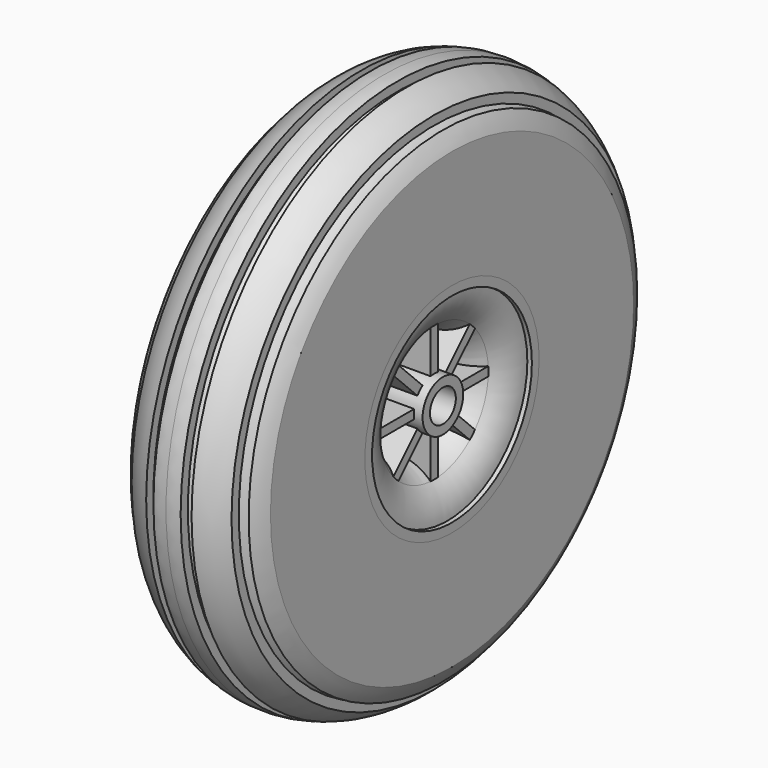
from build123d import *

# Parameters (mm, degrees)
F2_DEPTH = 0.635
F3_COUNT = 8
F3_ANGLE = 315


with BuildPart() as f1:
    # F0 (on Top) → F1 (revolve)
    with BuildSketch(Plane.XY):
        with BuildLine():
            Line((-8.255, 2.2606), (0, 2.2606))
            Line((0, 2.2606), (8.255, 2.2606))
            Line((8.255, 2.2606), (8.255, 3.556))
            Line((8.255, 3.556), (7.0301280605, 3.556))
            Line((7.0301280605, 3.556), (7.0301280605, 2.9083))
            Line((7.0301280605, 2.9083), (1.9207453588, 2.9083))
            Line((1.9207453588, 2.9083), (1.9207453588, 9.508256995))
            Line((1.9207453588, 9.508256995), (7.0301280605, 9.4798719395))
            ThreePointArc((7.0301280605, 9.4798719395), (8.4066350314, 11.5399602045), (8.89, 13.97))
            Line((8.89, 13.97), (9.525, 13.97))
            Line((9.525, 13.97), (9.525, 15.24))
            Line((9.525, 15.24), (8.255, 15.24))
            Line((8.255, 15.24), (8.255, 14.605))
            Line((8.255, 14.605), (0, 14.605))
            Line((0, 14.605), (-8.255, 14.605))
            Line((-8.255, 14.605), (-8.255, 15.24))
            Line((-8.255, 15.24), (-9.525, 15.24))
            Line((-9.525, 15.24), (-9.525, 13.97))
            Line((-9.525, 13.97), (-8.89, 13.97))
            ThreePointArc((-8.89, 13.97), (-8.4066350314, 11.5399602045), (-7.0301280605, 9.4798719395))
            Line((-7.0301280605, 9.4798719395), (-1.9207453588, 9.508256995))
            Line((-1.9207453588, 9.508256995), (-1.9207453588, 2.9083))
            Line((-1.9207453588, 2.9083), (-7.0301280605, 2.9083))
            Line((-7.0301280605, 2.9083), (-7.0301280605, 3.556))
            Line((-7.0301280605, 3.556), (-8.255, 3.556))
            Line((-8.255, 3.556), (-8.255, 2.2606))
        make_face()
        with BuildLine():
            Line((7.0301280605, 2.9083), (7.0301280605, 3.556))
            Line((7.0301280605, 3.556), (2.54, 3.556))
            Line((2.54, 3.556), (2.54, 7.62))
            ThreePointArc((2.54, 7.62), (4.9700397955, 8.1033649686), (7.0301280605, 9.4798719395))
            Line((7.0301280605, 9.4798719395), (1.9207453588, 9.508256995))
            Line((1.9207453588, 9.508256995), (1.9207453588, 2.9083))
            Line((1.9207453588, 2.9083), (7.0301280605, 2.9083))
        make_face()
        with BuildLine():
            Line((-2.54, 3.556), (-7.0301280605, 3.556))
            Line((-7.0301280605, 3.556), (-7.0301280605, 2.9083))
            Line((-7.0301280605, 2.9083), (-1.9207453588, 2.9083))
            Line((-1.9207453588, 2.9083), (-1.9207453588, 9.508256995))
            Line((-1.9207453588, 9.508256995), (-7.0301280605, 9.4798719395))
            ThreePointArc((-7.0301280605, 9.4798719395), (-4.9700397955, 8.1033649686), (-2.54, 7.62))
            Line((-2.54, 7.62), (-2.54, 3.556))
        make_face()
    revolve(axis=Axis((0.9157643653, 0, 0), (1, 0, 0)))

    # F0 (on Top) → F2 (join, symmetric)
    with BuildSketch(Plane.XY):
        with BuildLine():
            Line((7.0301280605, 2.9083), (7.0301280605, 3.556))
            Line((7.0301280605, 3.556), (2.54, 3.556))
            Line((2.54, 3.556), (2.54, 7.62))
            ThreePointArc((2.54, 7.62), (4.9700397955, 8.1033649686), (7.0301280605, 9.4798719395))
            Line((7.0301280605, 9.4798719395), (1.9207453588, 9.508256995))
            Line((1.9207453588, 9.508256995), (1.9207453588, 2.9083))
            Line((1.9207453588, 2.9083), (7.0301280605, 2.9083))
        make_face()
        with BuildLine():
            Line((2.54, 3.556), (7.0301280605, 3.556))
            Line((7.0301280605, 3.556), (7.0301280605, 9.4798719395))
            ThreePointArc((7.0301280605, 9.4798719395), (4.9700397955, 8.1033649686), (2.54, 7.62))
            Line((2.54, 7.62), (2.54, 3.556))
        make_face()
        with BuildLine():
            Line((-2.54, 3.556), (-7.0301280605, 3.556))
            Line((-7.0301280605, 3.556), (-7.0301280605, 2.9083))
            Line((-7.0301280605, 2.9083), (-1.9207453588, 2.9083))
            Line((-1.9207453588, 2.9083), (-1.9207453588, 9.508256995))
            Line((-1.9207453588, 9.508256995), (-7.0301280605, 9.4798719395))
            ThreePointArc((-7.0301280605, 9.4798719395), (-4.9700397955, 8.1033649686), (-2.54, 7.62))
            Line((-2.54, 7.62), (-2.54, 3.556))
        make_face()
        with BuildLine():
            Line((-7.0301280605, 9.4798719395), (-7.0301280605, 3.556))
            Line((-7.0301280605, 3.556), (-2.54, 3.556))
            Line((-2.54, 3.556), (-2.54, 7.62))
            ThreePointArc((-2.54, 7.62), (-4.9700397955, 8.1033649686), (-7.0301280605, 9.4798719395))
        make_face()
    extrude(amount=F2_DEPTH, both=True)

    # F3: F1 ×8 about axis
    f3_axis = Axis((0.9157643653, 0, 0), (1, 0, 0))


with BuildPart() as f1_1:
    add(f1.part)
    for i in range(1, F3_COUNT):
        add(f1.part.rotate(f3_axis, i * F3_ANGLE / (F3_COUNT - 1)))


with BuildPart() as f4:
    # F0 (on Top) → F4 (revolve)
    with BuildSketch(Plane.XY):
        with BuildLine():
            Line((8.255, 15.24), (9.525, 15.24))
            Line((9.525, 15.24), (9.525, 31.75))
            ThreePointArc((9.525, 31.75), (8.9591839228, 32.9007836702), (8.255, 33.9725))
            Line((8.255, 33.9725), (8.255, 32.7025))
            ThreePointArc((8.255, 32.7025), (7.6522635329, 33.4336386329), (6.985, 34.1064048083))
            Line((6.985, 34.1064048083), (6.985, 35.3764048083))
            ThreePointArc((6.985, 35.3764048083), (5.2001751556, 36.6938691388), (3.175, 37.599395271))
            Line((3.175, 37.599395271), (3.175, 36.329395271))
            ThreePointArc((3.175, 36.329395271), (2.5451365541, 36.511194074), (1.905, 36.6526294211))
            Line((1.905, 36.6526294211), (1.905, 37.9226294211))
            ThreePointArc((1.905, 37.9226294211), (0.9566197419, 38.0555616671), (0, 38.1))
            ThreePointArc((0, 38.1), (-0.9566197419, 38.0555616671), (-1.905, 37.9226294211))
            Line((-1.905, 37.9226294211), (-1.905, 36.6526294211))
            ThreePointArc((-1.905, 36.6526294211), (-2.5451365541, 36.511194074), (-3.175, 36.329395271))
            Line((-3.175, 36.329395271), (-3.175, 37.599395271))
            ThreePointArc((-3.175, 37.599395271), (-5.2001751556, 36.6938691388), (-6.985, 35.3764048083))
            Line((-6.985, 35.3764048083), (-6.985, 34.1064048083))
            ThreePointArc((-6.985, 34.1064048083), (-7.6522635329, 33.4336386329), (-8.255, 32.7025))
            Line((-8.255, 32.7025), (-8.255, 33.9725))
            ThreePointArc((-8.255, 33.9725), (-8.9591839228, 32.9007836702), (-9.525, 31.75))
            Line((-9.525, 31.75), (-9.525, 15.24))
            Line((-9.525, 15.24), (-8.255, 15.24))
            Line((-8.255, 15.24), (-8.255, 14.605))
            Line((-8.255, 14.605), (0, 14.605))
            Line((0, 14.605), (8.255, 14.605))
            Line((8.255, 14.605), (8.255, 15.24))
        make_face()
    revolve(axis=Axis((0.9157643653, 0, 0), (1, 0, 0)))


solid = Compound([f1_1.part, f4.part])
